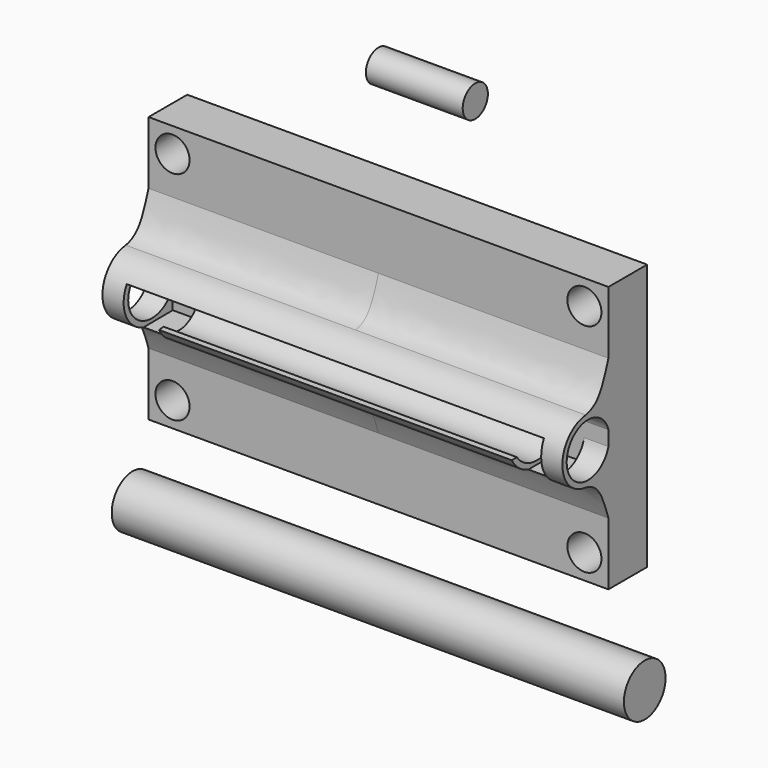
from build123d import *

# Parameters (mm, degrees)
F0_W      = 47.5
F0_H      = 55
F0_R      = 3.5231538004
F2_DEPTH  = 10
F3_DEPTH  = 47.5
F4_DEPTH  = 47.5
F5_W      = 5.5
F5_H      = 3.5
F6_DEPTH  = 116
F6_TAPER  = -3
F7_R      = 5.375
F8_DEPTH  = 55
F9_DEPTH  = 50.8
F10_R     = 3.25
F11_DEPTH = 25
F12_R     = 3.25
F13_DEPTH = 20


# Not quite as in the source:
# - an extrude ends at something that could not be found from the text; its depth is read off the source's solid


with BuildPart() as f2:
    # F0 (on Front) → F2 (new body)
    with BuildSketch(Plane.XZ):
        with Locations((-23.75, 0)):
            Rectangle(F0_W, F0_H)
        with Locations((-42.5404943526, -22.3999973387)):
            Circle(F0_R, mode=Mode.SUBTRACT)
        with Locations((-42.5404943526, 22.4092733115)):
            Circle(F0_R, mode=Mode.SUBTRACT)
        with Locations((23.75, 0)):
            Rectangle(F0_W, F0_H)
        with Locations((42.5404943526, -22.3999973387)):
            Circle(F0_R, mode=Mode.SUBTRACT)
        with Locations((42.5404943526, 22.4092733115)):
            Circle(F0_R, mode=Mode.SUBTRACT)
    extrude(amount=-F2_DEPTH)

    # F1 (on Right) → F3 (join)
    with BuildSketch(Plane.YZ):
        with BuildLine():
            ThreePointArc((0, -3.9765159025), (0.9884114859, -2.0964597633), (1.32962229, 0))
            ThreePointArc((1.32962229, 0), (0.9884114859, 2.0964597633), (0, 3.9765159025))
            Line((0, 3.9765159025), (0, 1.5348697397))
            ThreePointArc((0, 1.5348697397), (0.1636057764, 0.7751725864), (0.2185063777, 0))
            ThreePointArc((0.2185063777, 0), (0.1636057764, -0.7751725864), (0, -1.5348697397))
            Line((0, -1.5348697397), (0, -3.9765159025))
        make_face()
        with BuildLine():
            Line((0, -14.5392882731), (0, -14.5063873886))
            Line((0, -14.5063873886), (-0.0106325767, -14.5063873886))
            add(Edge.make_bspline(
                [(-0.0106325767, -14.5063873886), (-0.0070875742, -14.5173526167), (-0.0035433916, -14.5283196043), (0, -14.5392882731)],
                knots=[0.9975914602, 0.9975914602, 0.9975914602, 0.9975914602, 1, 1, 1, 1], degree=3))
        make_face()
        with BuildLine():
            Line((0, -14.5063873886), (0, -3.9765159025))
            ThreePointArc((0, -3.9765159025), (-2.5895292088, -6.0382266604), (-5.8538725864, -6.5862915155))
            add(Edge.make_bspline(
                [(-5.8538725864, -6.5862915155), (-4.8215552648, -6.8255458917), (-2.2801846921, -7.8765294876), (-0.8570999414, -11.8881360206), (-0.0106325767, -14.5063873886)],
                knots=[0.0813250355, 0.0813250355, 0.0813250355, 0.0813250355, 0.4224859886, 0.9975914602, 0.9975914602, 0.9975914602, 0.9975914602], degree=3))
            Line((-0.0106325767, -14.5063873886), (0, -14.5063873886))
        make_face()
        with BuildLine():
            Line((0, 1.5348697397), (0, 3.9765159025))
            ThreePointArc((0, 3.9765159025), (-2.5895292088, 6.0382266604), (-5.8538725864, 6.5862915155))
            ThreePointArc((-5.8538725864, 6.5862915155), (-11.8926095346, 0), (-5.8538725864, -6.5862915155))
            ThreePointArc((-5.8538725864, -6.5862915155), (-2.5895292088, -6.0382266604), (0, -3.9765159025))
            Line((0, -3.9765159025), (0, -1.5348697397))
            ThreePointArc((0, -1.5348697397), (-10.7814936223, 0), (0, 1.5348697397))
        make_face()
        with BuildLine():
            ThreePointArc((-5.8538725864, 6.5862915155), (-2.5895292088, 6.0382266604), (0, 3.9765159025))
            Line((0, 3.9765159025), (0, 14.5392882731))
            add(Edge.make_bspline(
                [(-5.8538725864, 6.5862915155), (-4.8215552648, 6.8255458917), (-2.2735043292, 7.8792921512), (-0.8496260973, 11.9092466626), (0, 14.5392882731)],
                knots=[0.0813250355, 0.0813250355, 0.0813250355, 0.0813250355, 0.4224859886, 1, 1, 1, 1], degree=3))
        make_face()
    extrude(amount=F3_DEPTH)

    # F4 (add): a face of the model
    f4_faces = [f2.faces().sort_by_distance(p)[0] for p in [
        (0, -0.31416521, -8.0370790064),
    ]]
    extrude(f4_faces, amount=F4_DEPTH)

    # F5 (on Front) → F6 (cut, through all)
    with BuildSketch(Plane.XZ):
        with Locations((-39.75, -4.25)):
            Rectangle(F5_W, F5_H)
        with Locations((39.75, -4.25)):
            Rectangle(F5_W, F5_H)
        Polygon((37, -2.5), (42.5, -2.5), (42.5, 2.5), (-42.5, 2.5), (-42.5, -2.5), (-37, -2.5), align=None)
    extrude(amount=F6_DEPTH, taper=F6_TAPER, mode=Mode.SUBTRACT)


with BuildPart() as f8:
    # F7 (on Right) → F8 (new body)
    with BuildSketch(Plane.YZ):
        with Locations((0, -43.3576591313)):
            Circle(F7_R)
    extrude(amount=F8_DEPTH)

    # F9 (add): a face of the model
    f9_faces = [f8.faces().sort_by_distance(p)[0] for p in [
        (0, 0, -43.3576591313),
    ]]
    extrude(f9_faces, amount=F9_DEPTH)

    # F10 (on Front) → F11 (cut)
    with BuildSketch(Plane.XZ):
        with Locations((41.2802435458, -43.0947579443)):
            Circle(F10_R)
    extrude(amount=-F11_DEPTH, mode=Mode.SUBTRACT)


with BuildPart() as f13:
    # F12 (on Right) → F13 (new body)
    with BuildSketch(Plane.YZ):
        with Locations((0, 52.3487925529)):
            Circle(F12_R)
    extrude(amount=F13_DEPTH)


solid = Compound([f2.part, f8.part, f13.part])
